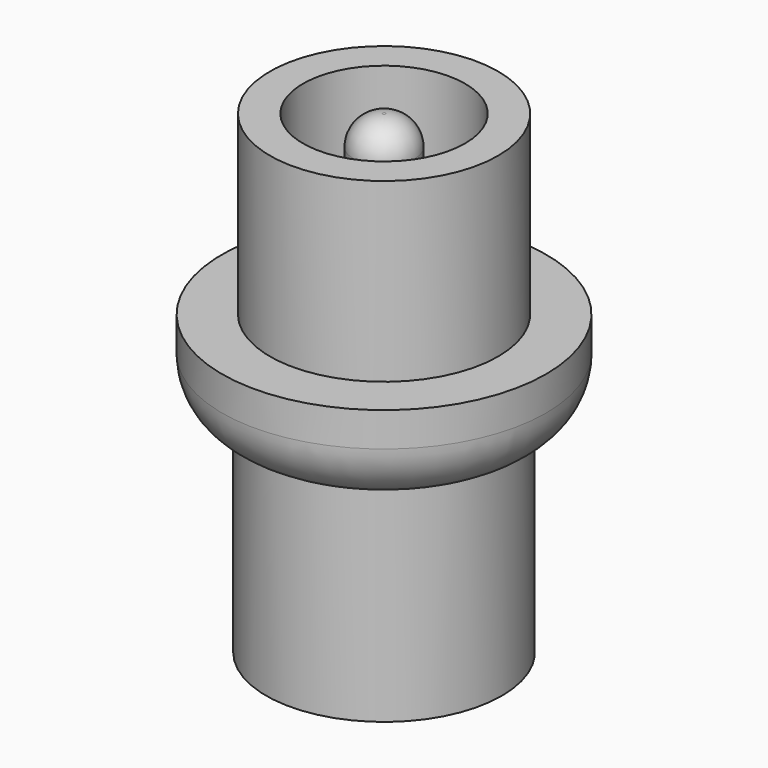
from build123d import *

# Parameters (mm, degrees)
F0_R     = 5.5
F1_DEPTH = 0.1
F2_R     = 3.875
F3_DEPTH = 6
F4_DEPTH = 3
F5_R     = 4
F6_DEPTH = 7
F7_R     = 2.75
F7_R_2   = 1.05
F8_DEPTH = 15
F9_R     = 1


# Not quite as in the source:
# - a fillet or chamfer that OpenCascade refuses, or shapes differently, is made with other operations: its cross-section is extruded or revolved along the edge and cut away or added


with BuildPart() as f1:
    # F0 (on Top) → F1 (new body)
    with BuildSketch(Plane.XY):
        Circle(F0_R)
    extrude(amount=F1_DEPTH)

    # F2 (on face) → F3 (join)
    with BuildSketch(Plane.XY.offset(0.1)):
        Circle(F2_R)
    extrude(amount=F3_DEPTH)

    # F0 (on Top) → F4 (join)
    with BuildSketch(Plane.XY):
        Circle(F0_R)
    extrude(amount=-F4_DEPTH)

    # F5 (on face) → F6 (join)
    with BuildSketch(Plane(origin=(0, 0, -3), x_dir=(1, 0, 0), z_dir=(0, 0, -1))):
        Circle(F5_R)
    extrude(amount=F6_DEPTH)

    # F7 (on face) → F8 (cut)
    with BuildSketch(Plane.XY.offset(6.1)):
        Circle(F7_R)
        Circle(F7_R_2, mode=Mode.SUBTRACT)
    extrude(amount=-F8_DEPTH, mode=Mode.SUBTRACT)

    # F9
    f9_edges = [f1.edges().sort_by_distance(p)[0] for p in [
        (-1.05, 0, 6.1),
    ]]
    fillet(f9_edges, radius=F9_R)

    # F10: fillet of radius 2 on 1 edges, made by hand

    # F10_s1 → F10_t2 (revolve, cut)
    with BuildSketch(Plane.XZ):
        with BuildLine():
            ThreePointArc((5.5, -1.0635083269), (5.0811388301, -2.2882531983), (4, -3))
            Line((4, -3), (5.5, -3))
            Line((5.5, -3), (5.5, -1.0635083269))
        make_face()
    revolve(axis=Axis((0, 0, -3), (0, 0, 1)), mode=Mode.SUBTRACT)


solid = f1.part
